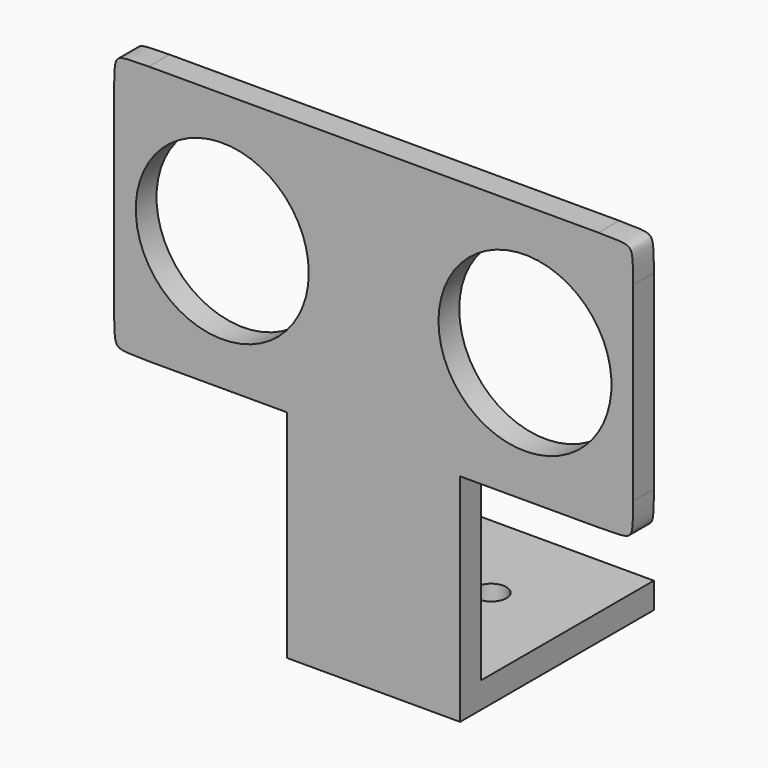
from build123d import *

# Parameters (mm, degrees)
F0_W        = 60
F0_H        = 30
F0_R        = 10
F1_DEPTH    = 3
F2_T1_DEPTH = 23
F3_W        = 20
F3_H        = 3
F4_DEPTH    = 25
F5_W        = 20
F5_H        = 3
F6_DEPTH    = 25
F7_R        = 1.75
F8_DEPTH    = 3.0010001


# Not quite as in the source:
# - a fillet or chamfer that OpenCascade refuses, or shapes differently, is made with other operations: its cross-section is extruded or revolved along the edge and cut away or added


with BuildPart() as f1:
    # F0 (on Front) → F1 (new body)
    with BuildSketch(Plane.XZ):
        Rectangle(F0_W, F0_H)
        with Locations((-17.5, 0)):
            Circle(F0_R, mode=Mode.SUBTRACT)
        with BuildLine():
            ThreePointArc((27.5, 0), (17.5, -10), (7.5, 0))
            ThreePointArc((7.5, 0), (17.5, 10), (27.5, 0))
        make_face(mode=Mode.SUBTRACT)
    extrude(amount=F1_DEPTH)

    # F2: fillet of radius 4 on 4 edges, made by hand

    # F2_s2 → F2_t1 (cut)
    with BuildSketch(Plane.XZ.offset(-10)):
        with BuildLine():
            add(Edge.make_bspline(
                [(30, -11), (30, -15), (26, -15)],
                knots=[0, 0, 0, 1, 1, 1], degree=2, weights=[1, 4, 1]))
            Line((26, -15), (30, -15))
            Line((30, -15), (30, -11))
        make_face()
        with BuildLine():
            add(Edge.make_bspline(
                [(-30, -11), (-30, -15), (-26, -15)],
                knots=[0, 0, 0, 1, 1, 1], degree=2, weights=[1, 4, 1]))
            Line((-26, -15), (-30, -15))
            Line((-30, -15), (-30, -11))
        make_face()
        with BuildLine():
            add(Edge.make_bspline(
                [(30, 11), (30, 15), (26, 15)],
                knots=[0, 0, 0, 1, 1, 1], degree=2, weights=[1, 4, 1]))
            Line((26, 15), (30, 15))
            Line((30, 15), (30, 11))
        make_face()
        with BuildLine():
            add(Edge.make_bspline(
                [(-30, 11), (-30, 15), (-26, 15)],
                knots=[0, 0, 0, 1, 1, 1], degree=2, weights=[1, 4, 1]))
            Line((-26, 15), (-30, 15))
            Line((-30, 15), (-30, 11))
        make_face()
    extrude(amount=F2_T1_DEPTH, mode=Mode.SUBTRACT)

    # F3 (on face) → F4 (join)
    with BuildSketch(Plane(origin=(0, 0, -15), x_dir=(1, 0, 0), z_dir=(0, 0, -1))):
        with Locations((0, 1.5)):
            Rectangle(F3_W, F3_H)
    extrude(amount=F4_DEPTH)

    # F5 (on face) → F6 (join)
    with BuildSketch(Plane(origin=(0, 0, 0), x_dir=(-1, 0, 0), z_dir=(0, 1, 0))):
        with Locations((0, -38.5)):
            Rectangle(F5_W, F5_H)
    extrude(amount=F6_DEPTH)

    # F7 (on face) → F8 (cut, through all)
    with BuildSketch(Plane.XY.offset(-37)):
        with Locations((0, 14)):
            Circle(F7_R)
    extrude(amount=-F8_DEPTH, mode=Mode.SUBTRACT)


solid = f1.part
